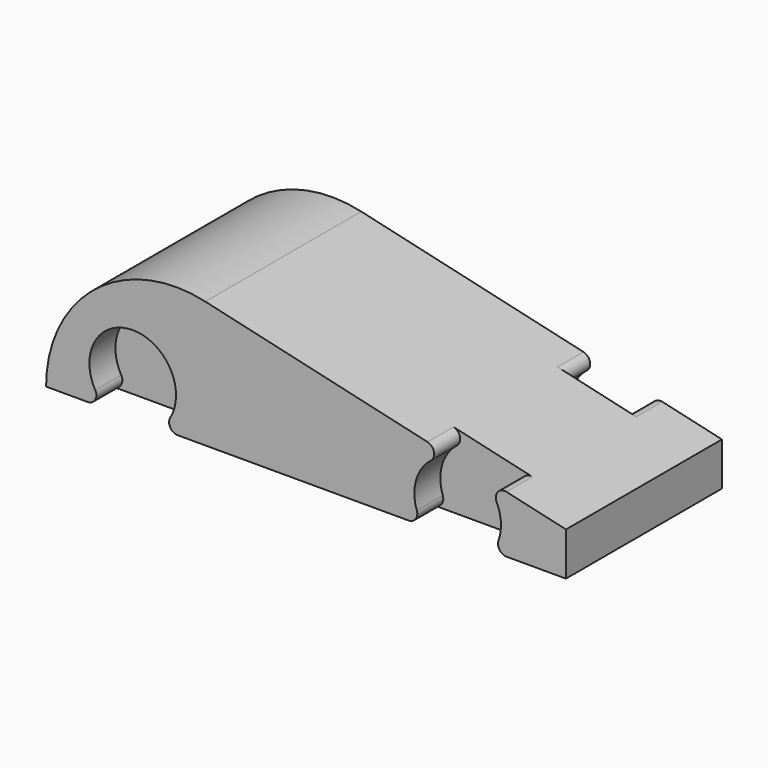
from build123d import *

# Parameters (mm, degrees)
F1_DEPTH = 28.575
F2_R     = 12.7
F3_DEPTH = 9.525
F4_R     = 2.54


# Not quite as in the source:
# - a pattern or mirror of a feature is missing from the dataset's text; its kind, count and spacing are read off the source's solid


with BuildPart() as f1:
    # F0 (on Front) → F1 (new body, symmetric)
    with BuildSketch(Plane.XZ):
        with BuildLine():
            Line((-152.4, 0), (0, 0))
            Line((0, 0), (0, 12.7))
            Line((0, 12.7), (-105.7247139353, 37.1224254179))
            ThreePointArc((-105.7247139353, 37.1224254179), (-138.0159397973, 29.8188564424), (-152.4, 0))
        make_face()
    extrude(amount=F1_DEPTH, both=True)

    # F2 (on face) → F3 (cut)
    with BuildSketch(Plane.XZ.offset(28.575)):
        with Locations((-127, 10.16)):
            Circle(F2_R)
        with Locations((-31.75, 7.62)):
            Circle(F2_R)
    f3 = extrude(amount=-F3_DEPTH, mode=Mode.SUBTRACT)

    # F3_copies: F3 across plane
    add(f3.mirror(Plane.ZX), mode=Mode.SUBTRACT)

    # F4
    f4_edges = [f1.edges().sort_by_distance(p)[0] for p in [
        (-25.256061, -23.8125, 18.534154),
        (-32.799092, -23.8125, 20.276595),
        (-41.91, -23.8125, 0),
        (-21.59, -23.8125, 0),
        (-134.62, -23.8125, 0),
        (-119.38, -23.8125, 0),
        (-21.59, 23.8125, 0),
        (-41.91, 23.8125, 0),
        (-119.38, 23.8125, 0),
        (-134.62, 23.8125, 0),
        (-32.799092, 23.8125, 20.276595),
        (-25.256061, 23.8125, 18.534154),
    ]]
    fillet(f4_edges, radius=F4_R)


solid = f1.part
